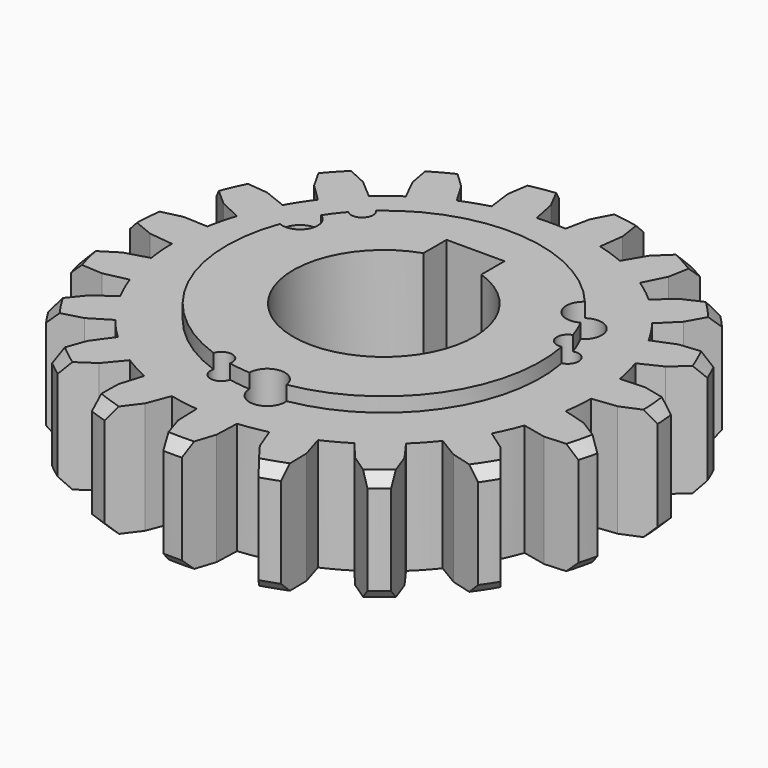
from build123d import *

# Parameters (mm, degrees)
F3_DEPTH        = 15.501
F5_SIZE         = 1.5
F7_DEPTH        = 17.501
F8_R            = 2.45
F8_R_2          = 1.5
F9_DEPTH        = 17.501
F9_COPIES_COUNT = 3


# Not quite as in the source:
# - a pattern or mirror of a feature is missing from the dataset's text; its kind, count and spacing are read off the source's solid


with BuildPart() as f1:
    # F0 (on Right) → F1 (revolve)
    with BuildSketch(Plane.YZ):
        Polygon((-36.5, 0), (-12.5, 0), (-12.5, 17.5), (-21.7, 17.5), (-21.7, 15.5), (-36.5, 15.5), align=None)
    revolve(axis=Axis((0, 0, 8.75), (0, 0, 1)))

    # F2 (on face) → F3 (cut, through all)
    with BuildSketch(Plane.XY.offset(15.5)):
        with BuildLine():
            Line((-2.6681709569, 32.2), (-2, 28.9))
            ThreePointArc((-2, 28.9), (0, 28.9691214917), (2, 28.9))
            Line((2, 28.9), (2.6681709569, 32.2))
            Line((2.6681709569, 32.2), (4.7396031012, 36.1909679678))
            ThreePointArc((4.7396031012, 36.1909679678), (2.3748335917, 36.422660054), (0, 36.5))
            ThreePointArc((0, 36.5), (-2.3748335917, 36.422660054), (-4.7396031012, 36.1909679678))
            Line((-4.7396031012, 36.1909679678), (-2.6681709569, 32.2))
        make_face()
        with BuildLine():
            Line((-7.9317208136, 31.3216688762), (-7.2683897572, 35.7689881089))
            ThreePointArc((-7.2683897572, 35.7689881089), (-11.851530626, 34.5223293221), (-16.2339864211, 32.6910948865))
            Line((-16.2339864211, 32.6910948865), (-12.9789250032, 29.5889614893))
            Line((-12.9789250032, 29.5889614893), (-11.2754491434, 26.6847193467))
            ThreePointArc((-11.2754491434, 26.6847193467), (-9.4062583717, 27.3994945838), (-7.4921801766, 27.9835172236))
            Line((-7.4921801766, 27.9835172236), (-7.9317208136, 31.3216688762))
        make_face()
        with BuildLine():
            ThreePointArc((16.2339864211, 32.6910948865), (11.851530626, 34.5223293221), (7.2683897572, 35.7689881089))
            Line((7.2683897572, 35.7689881089), (7.9317208136, 31.3216688762))
            Line((7.9317208136, 31.3216688762), (7.4921801766, 27.9835172236))
            ThreePointArc((7.4921801766, 27.9835172236), (9.4062583717, 27.3994945838), (11.2754491434, 26.6847193467))
            Line((11.2754491434, 26.6847193467), (12.9789250032, 29.5889614893))
            Line((12.9789250032, 29.5889614893), (16.2339864211, 32.6910948865))
        make_face()
        with BuildLine():
            Line((-17.6720875605, 27.0491489239), (-18.4887398047, 31.4708833755))
            ThreePointArc((-18.4887398047, 31.4708833755), (-22.4187640132, 28.803628593), (-25.969165416, 25.6486344198))
            Line((-25.969165416, 25.6486344198), (-21.8832111367, 23.7714998812))
            Line((-21.8832111367, 23.7714998812), (-19.3290284155, 21.5777352962))
            ThreePointArc((-19.3290284155, 21.5777352962), (-17.7932026956, 22.8607072907), (-16.1724663779, 24.0345861469))
            Line((-16.1724663779, 24.0345861469), (-17.6720875605, 27.0491489239))
        make_face()
        with BuildLine():
            ThreePointArc((25.969165416, 25.6486344198), (22.4187640132, 28.803628593), (18.4887398047, 31.4708833755))
            Line((18.4887398047, 31.4708833755), (17.6720875605, 27.0491489239))
            Line((17.6720875605, 27.0491489239), (16.1724663779, 24.0345861469))
            ThreePointArc((16.1724663779, 24.0345861469), (17.7932026956, 22.8607072907), (19.3290284155, 21.5777352962))
            Line((19.3290284155, 21.5777352962), (21.8832111367, 23.7714998812))
            Line((21.8832111367, 23.7714998812), (25.969165416, 25.6486344198))
        make_face()
        with BuildLine():
            Line((-25.4974094096, 19.8454339749), (-27.705548012, 23.7624201072))
            ThreePointArc((-27.705548012, 23.7624201072), (-30.5565764566, 19.9636077715), (-32.8901823849, 15.826746434))
            Line((-32.8901823849, 15.826746434), (-28.4161117905, 15.3780274082))
            Line((-28.4161117905, 15.3780274082), (-25.288007538, 14.1324688132))
            ThreePointArc((-25.288007538, 14.1324688132), (-24.2519774176, 15.8446076423), (-23.1002149055, 17.4811347263))
            Line((-23.1002149055, 17.4811347263), (-25.4974094096, 19.8454339749))
        make_face()
        with BuildLine():
            ThreePointArc((32.8901823849, 15.826746434), (30.5565764566, 19.9636077715), (27.705548012, 23.7624201072))
            Line((27.705548012, 23.7624201072), (25.4974094096, 19.8454339749))
            Line((25.4974094096, 19.8454339749), (23.1002149055, 17.4811347263))
            ThreePointArc((23.1002149055, 17.4811347263), (24.2519774176, 15.8446076423), (25.288007538, 14.1324688132))
            Line((25.288007538, 14.1324688132), (28.4161117905, 15.3780274082))
            Line((28.4161117905, 15.3780274082), (32.8901823849, 15.826746434))
        make_face()
        with BuildLine():
            Line((-30.5596913161, 10.4911583211), (-33.9200301964, 13.4789299084))
            ThreePointArc((-33.9200301964, 13.4789299084), (-35.3831097068, 8.9602202806), (-36.2470377487, 4.2897848949))
            Line((-36.2470377487, 4.2897848949), (-31.8696858104, 5.3181070507))
            Line((-31.8696858104, 5.3181070507), (-28.5066386599, 5.1557300465))
            ThreePointArc((-28.5066386599, 5.1557300465), (-28.0826740781, 7.1114989014), (-27.5246967114, 9.0333311102))
            Line((-27.5246967114, 9.0333311102), (-30.5596913161, 10.4911583211))
        make_face()
        with BuildLine():
            ThreePointArc((36.2470377487, 4.2897848949), (35.3831097068, 8.9602202806), (33.9200301964, 13.4789299084))
            Line((33.9200301964, 13.4789299084), (30.5596913161, 10.4911583211))
            Line((30.5596913161, 10.4911583211), (27.5246967114, 9.0333311102))
            ThreePointArc((27.5246967114, 9.0333311102), (28.0826740781, 7.1114989014), (28.5066386599, 5.1557300465))
            Line((28.5066386599, 5.1557300465), (31.8696858104, 5.3181070507))
            Line((31.8696858104, 5.3181070507), (36.2470377487, 4.2897848949))
        make_face()
        with BuildLine():
            Line((-32.310356486, 2.8761e-06), (-36.4587507855, 1.7347885069))
            ThreePointArc((-36.4587507855, 1.7347885069), (-36.3753339947, -3.0141461097), (-35.6759641417, -7.7120414005))
            Line((-35.6759641417, -7.7120414005), (-31.8696848636, -5.3181127245))
            Line((-31.8696848636, -5.3181127245), (-28.6361331569, -4.3797120702))
            ThreePointArc((-28.6361331569, -4.3797120702), (-28.8701772546, -2.3922510917), (-28.9664505388, -0.3933740981))
            Line((-28.9664505388, -0.3933740981), (-32.310356486, 2.8761e-06))
        make_face()
        with BuildLine():
            ThreePointArc((36.5, 0), (36.4896862392, 0.8676394213), (36.4587507855, 1.7347885069))
            Line((36.4587507855, 1.7347885069), (32.310356486, 2.8761e-06))
            Line((32.310356486, 2.8761e-06), (28.9664505388, -0.3933740981))
            ThreePointArc((28.9664505388, -0.3933740981), (28.8701772546, -2.3922510917), (28.6361331569, -4.3797120702))
            Line((28.6361331569, -4.3797120702), (31.8696848636, -5.3181127245))
            Line((31.8696848636, -5.3181127245), (35.6759641417, -7.7120414005))
            ThreePointArc((35.6759641417, -7.7120414005), (36.2934063651, -3.8779703989), (36.5, 0))
        make_face()
        with BuildLine():
            Line((-30.5596931839, -10.4911528805), (-35.0466000111, -10.1973441474))
            ThreePointArc((-35.0466000111, -10.1973441474), (-33.4257264229, -14.6618829998), (-31.2388462503, -18.8781483454))
            Line((-31.2388462503, -18.8781483454), (-28.4161090527, -15.3780324671))
            Line((-28.4161090527, -15.3780324671), (-25.662458291, -13.4405444258))
            ThreePointArc((-25.662458291, -13.4405444258), (-26.5291487587, -11.6367635594), (-27.2692399896, -9.7774511192))
            Line((-27.2692399896, -9.7774511192), (-30.5596931839, -10.4911528805))
        make_face()
        with BuildLine():
            Line((-25.4974129427, -19.8454294356), (-29.8366063215, -21.0244363352))
            ThreePointArc((-29.8366063215, -21.0244363352), (-26.8539227396, -24.7207773643), (-23.416514647, -27.9985149925))
            Line((-23.416514647, -27.9985149925), (-21.8832069046, -23.7715037771))
            Line((-21.8832069046, -23.7715037771), (-19.9078578752, -21.0448852413))
            ThreePointArc((-19.9078578752, -21.0448852413), (-21.3132753526, -19.6202521325), (-22.6169841617, -18.1019895986))
            Line((-22.6169841617, -18.1019895986), (-25.4974129427, -19.8454294356))
        make_face()
        with BuildLine():
            ThreePointArc((31.2388462503, -18.8781483454), (33.4257264229, -14.6618829998), (35.0466000111, -10.1973441474))
            Line((35.0466000111, -10.1973441474), (30.5596931839, -10.4911528805))
            Line((30.5596931839, -10.4911528805), (27.2692399896, -9.7774511192))
            ThreePointArc((27.2692399896, -9.7774511192), (26.5291487587, -11.6367635594), (25.662458291, -13.4405444258))
            Line((25.662458291, -13.4405444258), (28.4161090527, -15.3780324671))
            Line((28.4161090527, -15.3780324671), (31.2388462503, -18.8781483454))
        make_face()
        with BuildLine():
            Line((-17.6720923761, -27.0491457777), (-21.3933533744, -29.5732046183))
            ThreePointArc((-21.3933533744, -29.5732046183), (-17.3720798459, -32.100791919), (-13.0566403371, -34.0848080984))
            Line((-13.0566403371, -34.0848080984), (-12.9789197355, -29.5889638))
            Line((-12.9789197355, -29.5889638), (-11.9959321564, -26.3686861959))
            ThreePointArc((-11.9959321564, -26.3686861959), (-13.7877778525, -25.4775819474), (-15.5138271612, -24.4648966238))
            Line((-15.5138271612, -24.4648966238), (-17.6720923761, -27.0491457777))
        make_face()
        with BuildLine():
            ThreePointArc((23.416514647, -27.9985149925), (26.8539227396, -24.7207773643), (29.8366063215, -21.0244363352))
            Line((29.8366063215, -21.0244363352), (25.4974129427, -19.8454294356))
            Line((25.4974129427, -19.8454294356), (22.6169841617, -18.1019895986))
            ThreePointArc((22.6169841617, -18.1019895986), (21.3132753526, -19.6202521325), (19.9078578752, -21.0448852413))
            Line((19.9078578752, -21.0448852413), (21.8832069046, -23.7715037771))
            Line((21.8832069046, -23.7715037771), (23.416514647, -27.9985149925))
        make_face()
        with BuildLine():
            Line((-7.9317263898, -31.3216674641), (-10.631798637, -34.9172573055))
            ThreePointArc((-10.631798637, -34.9172573055), (-6.0077025452, -36.0021875742), (-1.281876452, -36.4774833666))
            Line((-1.281876452, -36.4774833666), (-2.6681652243, -32.200000475))
            Line((-2.6681652243, -32.200000475), (-2.7840610523, -28.8350308489))
            ThreePointArc((-2.7840610523, -28.8350308489), (-4.7681606827, -28.574020433), (-6.7295062659, -28.1766524878))
            Line((-6.7295062659, -28.1766524878), (-7.9317263898, -31.3216674641))
        make_face()
        with BuildLine():
            ThreePointArc((13.0566403371, -34.0848080984), (17.3720798459, -32.100791919), (21.3933533744, -29.5732046183))
            Line((21.3933533744, -29.5732046183), (17.6720923761, -27.0491457777))
            Line((17.6720923761, -27.0491457777), (15.5138271612, -24.4648966238))
            ThreePointArc((15.5138271612, -24.4648966238), (13.7877778525, -25.4775819474), (11.9959321564, -26.3686861959))
            Line((11.9959321564, -26.3686861959), (12.9789197355, -29.5889638))
            Line((12.9789197355, -29.5889638), (13.0566403371, -34.0848080984))
        make_face()
        with BuildLine():
            Line((2.6681652243, -32.200000475), (1.281876452, -36.4774833666))
            ThreePointArc((1.281876452, -36.4774833666), (6.0077025452, -36.0021875742), (10.631798637, -34.9172573055))
            Line((10.631798637, -34.9172573055), (7.9317263898, -31.3216674641))
            Line((7.9317263898, -31.3216674641), (6.7295062659, -28.1766524878))
            ThreePointArc((6.7295062659, -28.1766524878), (4.7681606827, -28.574020433), (2.7840610523, -28.8350308489))
            Line((2.7840610523, -28.8350308489), (2.6681652243, -32.200000475))
        make_face()
    extrude(amount=-F3_DEPTH, mode=Mode.SUBTRACT)

    # F5
    f5_edges = [f1.edges().sort_by_distance(p)[0] for p in [
        (0, -36.5, 0),
        (11.851531, -34.522329, 0),
        (22.418764, -28.803629, 0),
        (30.556576, -19.963608, 0),
        (35.38311, -8.96022, 0),
        (36.375334, 3.014146, 0),
        (33.425726, 14.661883, 0),
        (26.853923, 24.720777, 0),
        (17.37208, 32.100792, 0),
        (6.007703, 36.002188, 0),
        (-6.007703, 36.002188, 0),
        (-17.37208, 32.100792, 0),
        (-26.853923, 24.720777, 0),
        (-33.425726, 14.661883, 0),
        (-36.375334, 3.014146, 0),
        (-35.38311, -8.96022, 0),
        (-30.556576, -19.963608, 0),
        (-22.418764, -28.803629, 0),
        (-11.851531, -34.522329, 0),
        (0, -36.5, 15.5),
        (-11.851531, -34.522329, 15.5),
        (-22.418764, -28.803629, 15.5),
        (-30.556576, -19.963608, 15.5),
        (-35.38311, -8.96022, 15.5),
        (-36.375334, 3.014146, 15.5),
        (-33.425726, 14.661883, 15.5),
        (-26.853923, 24.720777, 15.5),
        (-17.37208, 32.100792, 15.5),
        (-6.007703, 36.002188, 15.5),
        (6.007703, 36.002188, 15.5),
        (17.37208, 32.100792, 15.5),
        (26.853923, 24.720777, 15.5),
        (33.425726, 14.661883, 15.5),
        (36.375334, 3.014146, 15.5),
        (35.38311, -8.96022, 15.5),
        (30.556576, -19.963608, 15.5),
        (22.418764, -28.803629, 15.5),
        (11.851531, -34.522329, 15.5),
    ]]
    chamfer(f5_edges, length=F5_SIZE)

    # F6 (on face) → F7 (cut, through all)
    with BuildSketch(Plane.XY.offset(17.5)):
        Polygon((-4, 15.8427192823), (-4, 11.8427192823), (4, 11.8427192823), (4, 15.8427192823), (0, 15.8427192823), align=None)
    extrude(amount=-F7_DEPTH, mode=Mode.SUBTRACT)

    # F8 (on face) → F9 (cut, through all)
    with BuildSketch(Plane.XY.offset(17.5)):
        with Locations((18.1458966351, 11.900270388)):
            Circle(F8_R)
        with Locations((20.9774100604, 5.5532213318)):
            Circle(F8_R_2)
    f9 = extrude(amount=-F9_DEPTH, mode=Mode.SUBTRACT)

    # F9_copies: F9 ×3 about axis
    f9_copies_axis = Axis((0, 0, 0), (0, 0, 1))
    for i in range(1, F9_COPIES_COUNT):
        add(f9.rotate(f9_copies_axis, i * 360 / F9_COPIES_COUNT), mode=Mode.SUBTRACT)


solid = f1.part
